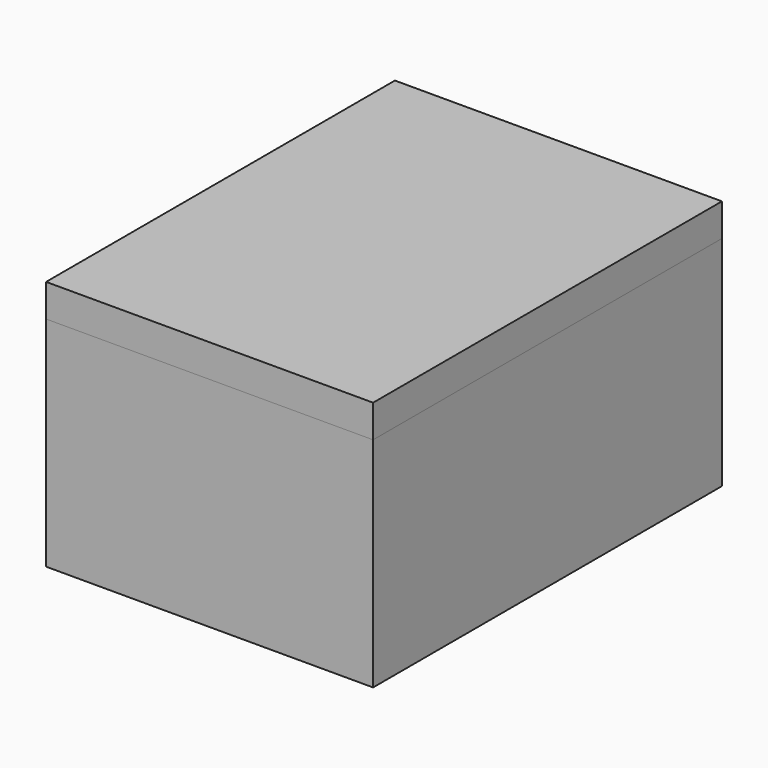
from build123d import *

# Parameters (mm, degrees)
F0_W     = 60
F0_H     = 80
F1_DEPTH = 40
F2_T     = -3
F3_W     = 60
F3_H     = 80
F3_W_2   = 54
F3_H_2   = 74
F4_DEPTH = 3
F5_DEPTH = 3
F6_DEPTH = 4


# Not quite as in the source:
# - the program builds the solid bodies; features that only make, move or delete a surface that nothing else refers to are left out


with BuildPart() as f1:
    # F0 (on Top) → F1 (new body)
    with BuildSketch(Plane.XY):
        Rectangle(F0_W, F0_H)
    extrude(amount=F1_DEPTH)

    # F2
    f2_openings = [f1.faces().sort_by_distance(p)[0] for p in [
        (0, 0, 40),
    ]]
    offset(amount=F2_T, openings=f2_openings)


with BuildPart() as f4:
    # F3 (on face) → F4 (new body)
    with BuildSketch(Plane.XY.offset(40)):
        Rectangle(F3_W, F3_H)
        Rectangle(F3_W_2, F3_H_2, mode=Mode.SUBTRACT)
        Rectangle(F3_W_2, F3_H_2)
    extrude(amount=F4_DEPTH)

    # F5 (add): a face of the model
    f5_faces = [f4.faces().sort_by_distance(p)[0] for p in [
        (0, 0, 43),
    ]]
    extrude(f5_faces, amount=F5_DEPTH)

    # F3 (on face) → F6 (join)
    with BuildSketch(Plane.XY.offset(40)):
        Rectangle(F3_W_2, F3_H_2)
    extrude(amount=-F6_DEPTH)


solid = Compound([f1.part, f4.part])
